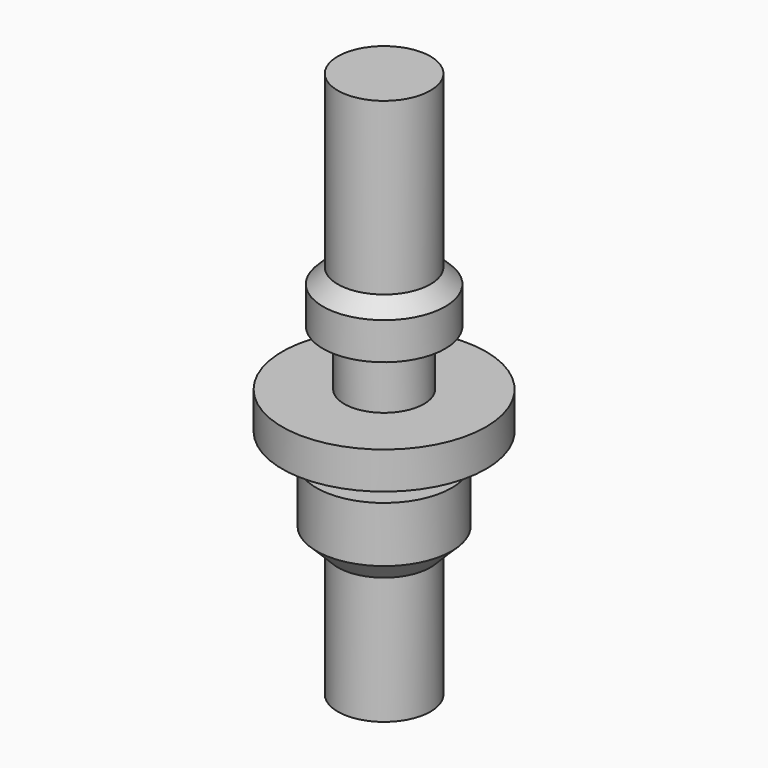
from build123d import *

# Parameters (mm, degrees)
F0_R         = 5.5
F1_DEPTH     = 2
F2_R         = 2.15
F3_DEPTH     = 3
F4_R         = 3.3
F5_DEPTH     = 12
F6_R         = 5
F6_R_2       = 2.5
F7_DEPTH     = 7
F8_S5_R      = 2.5
F8_T6_DEPTH  = 6
F9_R         = 2.5
F10_DEPTH    = 1.5
F11_R        = 3.65
F12_DEPTH    = 11
F13_R        = 5
F13_R_2      = 2.5
F14_DEPTH    = 5
F15_S5_R     = 2.5
F15_T6_DEPTH = 7


# Not quite as in the source:
# - a fillet or chamfer that OpenCascade refuses, or shapes differently, is made with other operations: its cross-section is extruded or revolved along the edge and cut away or added


with BuildPart() as f1:
    # F0 (on Top) → F1 (new body)
    with BuildSketch(Plane.XY):
        Circle(F0_R)
    extrude(amount=F1_DEPTH)

    # F2 (on face) → F3 (join)
    with BuildSketch(Plane.XY.offset(2)):
        Circle(F2_R)
    extrude(amount=F3_DEPTH)

    # F4 (on face) → F5 (join)
    with BuildSketch(Plane.XY.offset(5)):
        Circle(F4_R)
    extrude(amount=F5_DEPTH)

    # F6 (on face) → F7 (cut)
    with BuildSketch(Plane.XY.offset(17)):
        Circle(F6_R)
        Circle(F6_R_2, mode=Mode.SUBTRACT)
    extrude(amount=-F7_DEPTH, mode=Mode.SUBTRACT)

    # F8: chamfer of 3 on 1 edges, made by hand


with BuildPart() as f8_tool2:
    # F8_s3 → F8_t4 (revolve)
    with BuildSketch(Plane.XZ):
        Polygon((3.3, 7), (0.3, 10), (3.3, 10), align=None)
    revolve(axis=Axis((0, 0, 10), (0, 0, -1)))

    # F8_s5 → F8_t6 (cut, symmetric)
    with BuildSketch(Plane.XY.offset(8.5)):
        Circle(F8_S5_R)
    extrude(amount=F8_T6_DEPTH, both=True, mode=Mode.SUBTRACT)


with BuildPart() as f1_1:
    add(f1.part)

    # F8_t1: cut F8_tool2
    add(f8_tool2.part, mode=Mode.SUBTRACT)

    # F9 (on face) → F10 (join)
    with BuildSketch(Plane(origin=(0, 0, 0), x_dir=(1, 0, 0), z_dir=(0, 0, -1))):
        Circle(F9_R)
    extrude(amount=F10_DEPTH)

    # F11 (on face) → F12 (join)
    with BuildSketch(Plane(origin=(0, 0, -1.5), x_dir=(1, 0, 0), z_dir=(0, 0, -1))):
        Circle(F11_R)
    extrude(amount=F12_DEPTH)

    # F13 (on face) → F14 (cut)
    with BuildSketch(Plane(origin=(0, 0, -12.5), x_dir=(1, 0, 0), z_dir=(0, 0, -1))):
        Circle(F13_R)
        Circle(F13_R_2, mode=Mode.SUBTRACT)
    extrude(amount=-F14_DEPTH, mode=Mode.SUBTRACT)

    # F15: chamfer of 3 on 1 edges, made by hand


with BuildPart() as f15_tool2:
    # F15_s3 → F15_t4 (revolve)
    with BuildSketch(Plane.XZ):
        Polygon((3.65, -4.5), (0.65, -7.5), (3.65, -7.5), align=None)
    revolve(axis=Axis((0, 0, -7.5), (0, 0, 1)))

    # F15_s5 → F15_t6 (cut, symmetric)
    with BuildSketch(Plane.XY.offset(-6)):
        Circle(F15_S5_R)
    extrude(amount=F15_T6_DEPTH, both=True, mode=Mode.SUBTRACT)


with BuildPart() as f1_2:
    add(f1_1.part)

    # F15_t1: cut F15_tool2
    add(f15_tool2.part, mode=Mode.SUBTRACT)


solid = f1_2.part
